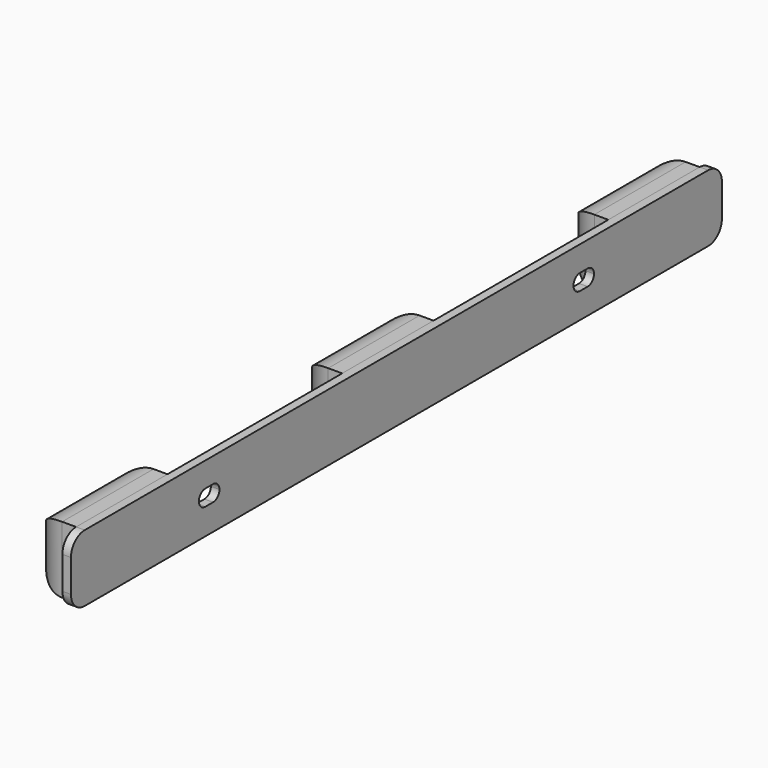
from build123d import *

# Parameters (mm, degrees)
F0_W     = 361.95
F0_H     = 29.718
F1_DEPTH = 3.81
F2_R     = 7.62
F4_DEPTH = 3.81
F5_W     = 50.8
F5_H     = 29.718
F6_DEPTH = 21.082
F7_R     = 14.85899
F7_2_R   = 14.85899
F7_3_R   = 14.85899


# Not quite as in the source:
# - a fillet or chamfer is up to 0.001 mm smaller than in the source, because OpenCascade refuses the exact size


with BuildPart() as f1:
    # F0 (on Right) → F1 (new body)
    with BuildSketch(Plane.YZ):
        Rectangle(F0_W, F0_H)
    extrude(amount=F1_DEPTH)

    # F2
    f2_edges = [f1.edges().sort_by_distance(p)[0] for p in [
        (1.905, 180.975, 14.859),
        (1.905, 180.975, -14.859),
        (1.905, -180.975, 14.859),
        (1.905, -180.975, -14.859),
    ]]
    fillet(f2_edges, radius=F2_R)

    # F3 (on face) → F4 (cut, through all)
    with BuildSketch(Plane(origin=(0, 0, 0), x_dir=(0, -1, 0), z_dir=(-1, 0, 0))):
        with BuildLine():
            Line((-101.981, 3.6386192348), (-106.299, 3.6386192348))
            ThreePointArc((-106.299, 3.6386192348), (-108.8134717139, 2.5970909487), (-109.855, 0.0826192348))
            ThreePointArc((-109.855, 0.0826192348), (-108.8134717139, -2.4318524791), (-106.299, -3.4733807652))
            Line((-106.299, -3.4733807652), (-101.981, -3.4733807652))
            ThreePointArc((-101.981, -3.4733807652), (-99.4665282861, -2.4318524791), (-98.425, 0.0826192348))
            ThreePointArc((-98.425, 0.0826192348), (-99.4665282861, 2.5970909487), (-101.981, 3.6386192348))
        make_face()
        with BuildLine():
            Line((106.299, 3.8625788135), (101.981, 3.8625788135))
            ThreePointArc((101.981, 3.8625788135), (99.4665282861, 2.8210505274), (98.425, 0.3065788135))
            ThreePointArc((98.425, 0.3065788135), (99.4665282861, -2.2078929004), (101.981, -3.2494211865))
            Line((101.981, -3.2494211865), (106.299, -3.2494211865))
            ThreePointArc((106.299, -3.2494211865), (108.8134717139, -2.2078929004), (109.855, 0.3065788135))
            ThreePointArc((109.855, 0.3065788135), (108.8134717139, 2.8210505274), (106.299, 3.8625788135))
        make_face()
    extrude(amount=-F4_DEPTH, mode=Mode.SUBTRACT)


with BuildPart() as f6:
    # F5 (on face) → F6 (new body)
    with BuildSketch(Plane(origin=(0, 0, 0), x_dir=(0, -1, 0), z_dir=(-1, 0, 0))):
        with Locations((-147.955, 0)):
            Rectangle(F5_W, F5_H)
    extrude(amount=F6_DEPTH)

    # F7 (radius 14.859 in the source; OpenCascade refuses exactly that, so slightly less here)
    f7_edges = [f6.edges().sort_by_distance(p)[0] for p in [
        (-21.082, 147.955, 14.859),
        (-21.082, 173.355, 0),
        (-21.082, 147.955, -14.859),
        (-21.082, 122.555, 0),
    ]]
    fillet(f7_edges, radius=F7_R)


with BuildPart() as f6b:
    # F5 (on face) → F6, piece 2 (new body)
    with BuildSketch(Plane(origin=(0, 0, 0), x_dir=(0, -1, 0), z_dir=(-1, 0, 0))):
        Rectangle(F5_W, F5_H)
    extrude(amount=F6_DEPTH)

    # F7#2 (radius 14.859 in the source; OpenCascade refuses exactly that, so slightly less here)
    f7_2_edges = [f6b.edges().sort_by_distance(p)[0] for p in [
        (-21.082, 0, 14.859),
        (-21.082, 25.4, 0),
        (-21.082, 0, -14.859),
        (-21.082, -25.4, 0),
    ]]
    fillet(f7_2_edges, radius=F7_2_R)


with BuildPart() as f6c:
    # F5 (on face) → F6, piece 3 (new body)
    with BuildSketch(Plane(origin=(0, 0, 0), x_dir=(0, -1, 0), z_dir=(-1, 0, 0))):
        with Locations((147.955, 0)):
            Rectangle(F5_W, F5_H)
    extrude(amount=F6_DEPTH)

    # F7#3 (radius 14.859 in the source; OpenCascade refuses exactly that, so slightly less here)
    f7_3_edges = [f6c.edges().sort_by_distance(p)[0] for p in [
        (-21.082, -147.955, 14.859),
        (-21.082, -122.555, 0),
        (-21.082, -147.955, -14.859),
        (-21.082, -173.355, 0),
    ]]
    fillet(f7_3_edges, radius=F7_3_R)


solid = Compound([f1.part, f6.part, f6b.part, f6c.part])
